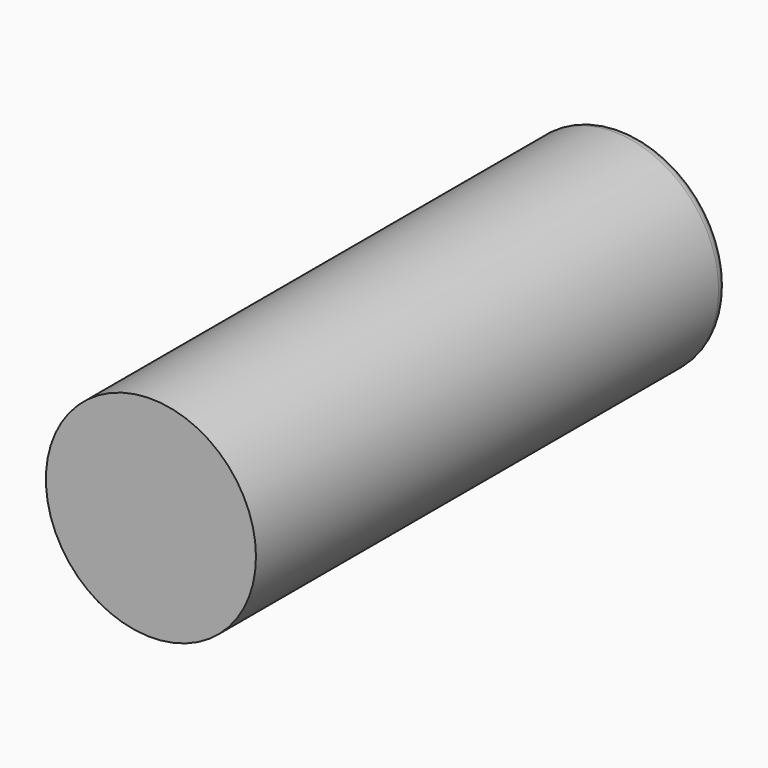
from build123d import *

# Parameters (mm, degrees)
F0_R     = 89
F1_DEPTH = 500
F2_R     = 10


# Not quite as in the source:
# - a feature names something its author has since deleted; it is built from what else it names


with BuildPart() as f1:
    # F0 (on Front) → F1 (new body)
    with BuildSketch(Plane.XZ):
        Circle(F0_R)
    extrude(amount=-F1_DEPTH)

    # F2
    f2_edges = [f1.edges().sort_by_distance(p)[0] for p in [
        (-89, 500, 0),
    ]]
    fillet(f2_edges, radius=F2_R)


solid = f1.part
